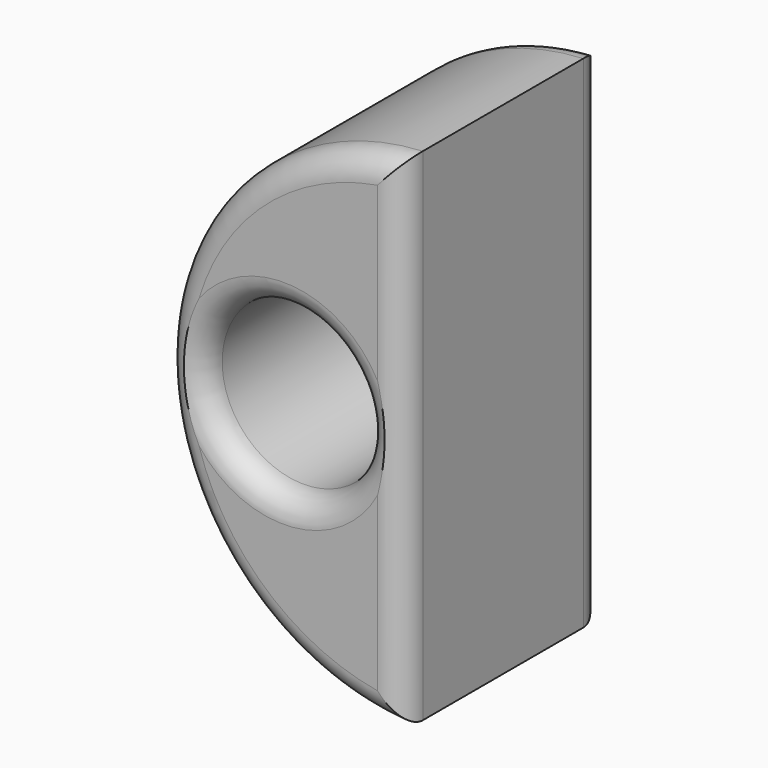
from build123d import *

# Parameters (mm, degrees)
F1_DEPTH    = 20
F2_R        = 6.5
F3_DEPTH    = 20
F4_T1_DEPTH = 49.9499687109
F4_T4_ANGLE = 202.9591024792
F4_T6_ANGLE = 202.9591024792


# Not quite as in the source:
# - a fillet or chamfer that OpenCascade refuses, or shapes differently, is made with other operations: its cross-section is extruded or revolved along the edge and cut away or added


with BuildPart() as f1:
    # F0 (on Front) → F1 (new body)
    with BuildSketch(Plane.XZ):
        with BuildLine():
            Line((-1, 0), (-1, 19.9749843554))
            ThreePointArc((-1, 19.9749843554), (-20, 0), (-1, -19.9749843554))
            Line((-1, -19.9749843554), (-1, 0))
        make_face()
    extrude(amount=F1_DEPTH)

    # F2 (on face) → F3 (cut)
    with BuildSketch(Plane.XZ.offset(20)):
        with Locations((-10.5, 0)):
            Circle(F2_R)
    extrude(amount=-F3_DEPTH, mode=Mode.SUBTRACT)

    # F4: fillet of radius 2 on 6 edges, made by hand

    # F4_s2 → F4_t1 (cut)
    with BuildSketch(Plane.XY.offset(-24.9749843554)):
        with BuildLine():
            ThreePointArc((-1, -18), (-1.5857864376, -19.4142135624), (-3, -20))
            Line((-3, -20), (-1, -20))
            Line((-1, -20), (-1, -18))
        make_face()
        with BuildLine():
            ThreePointArc((-1, -2), (-1.5857864376, -0.5857864376), (-3, 0))
            Line((-3, 0), (-1, 0))
            Line((-1, 0), (-1, -2))
        make_face()
    extrude(amount=F4_T1_DEPTH, mode=Mode.SUBTRACT)

    # F4_s3 → F4_t4 (revolve, cut)
    with BuildSketch(Plane(origin=(0, 0, 0), x_dir=(0, 1, 0), z_dir=(0.9799957963, 0, -0.1990181884))):
        with BuildLine():
            ThreePointArc((-18, 20), (-19.4142135624, 19.4142135624), (-20, 18))
            Line((-20, 18), (-20, 20))
            Line((-20, 20), (-18, 20))
        make_face()
    revolve(axis=Axis((0, -20, 0), (0, -1, 0)), revolution_arc=F4_T4_ANGLE, mode=Mode.SUBTRACT)

    # F4_s5 → F4_t6 (revolve, cut)
    with BuildSketch(Plane(origin=(0, 0, 0), x_dir=(0, 1, 0), z_dir=(0.9799957963, 0, -0.1990181884))):
        with BuildLine():
            ThreePointArc((-2, 20), (-0.5857864376, 19.4142135624), (0, 18))
            Line((0, 18), (0, 20))
            Line((0, 20), (-2, 20))
        make_face()
    revolve(axis=Axis((0, 0, 0), (0, -1, 0)), revolution_arc=F4_T6_ANGLE, mode=Mode.SUBTRACT)

    # F4_s7 → F4_t8 (revolve, cut)
    with BuildSketch(Plane.XY):
        with BuildLine():
            ThreePointArc((-2, 0), (-3.4142135624, -0.5857864376), (-4, -2))
            Line((-4, -2), (-4, 0))
            Line((-4, 0), (-2, 0))
        make_face()
    revolve(axis=Axis((-10.5, 0, 0), (0, -1, 0)), mode=Mode.SUBTRACT)

    # F4_s9 → F4_t10 (revolve, cut)
    with BuildSketch(Plane.XY):
        with BuildLine():
            ThreePointArc((-2, -20), (-3.4142135624, -19.4142135624), (-4, -18))
            Line((-4, -18), (-4, -20))
            Line((-4, -20), (-2, -20))
        make_face()
    revolve(axis=Axis((-10.5, -20, 0), (0, -1, 0)), mode=Mode.SUBTRACT)


solid = f1.part
